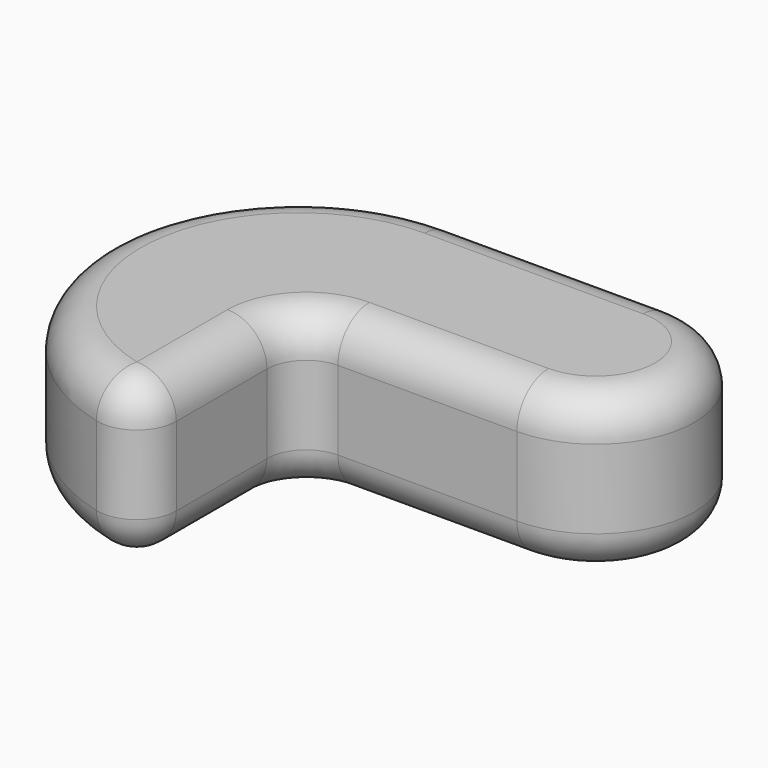
from build123d import *

# Parameters (mm, degrees)
F0_W     = 27.7
F0_H     = 25
F1_DEPTH = 10
F2_DEPTH = 10
F3_R     = 5


# Not quite as in the source:
# - a feature names something its author has since deleted; it is built from what else it names


with BuildPart() as f1:
    # F0 (on Top) → F1 (new body)
    with BuildSketch(Plane.XY):
        with BuildLine():
            Line((-18, 25), (-18, 50))
            ThreePointArc((-18, 50), (-43, 25), (-18, 0))
            Line((-18, 0), (-18, 25))
        make_face()
        with BuildLine():
            ThreePointArc((9.7, 25), (22.2, 37.5), (9.7, 50))
            Line((9.7, 50), (9.7, 25))
        make_face()
        with Locations((-4.15, 37.5)):
            Rectangle(F0_W, F0_H)
    extrude(amount=F1_DEPTH)

    # F2 (add): a face of the model
    f2_faces = [f1.faces().sort_by_distance(p)[0] for p in [
        (-14.2102397427, 31.107363361, 10),
    ]]
    extrude(f2_faces, amount=F2_DEPTH)

    # F3
    f3_edges = [f1.edges().sort_by_distance(p)[0] for p in [
        (-4.15, 25, 20),
        (9.7, 25, 10),
        (-4.15, 25, 0),
        (-18, 25, 10),
        (-4.15, 50, 20),
        (22.2, 37.5, 20),
        (-43, 25, 20),
        (-18, 12.5, 20),
        (-18, 50, 10),
        (-18, 0, 10),
        (-43, 25, 0),
        (-18, 12.5, 0),
        (22.2, 37.5, 0),
        (-4.15, 50, 0),
    ]]
    fillet(f3_edges, radius=F3_R)


solid = f1.part
